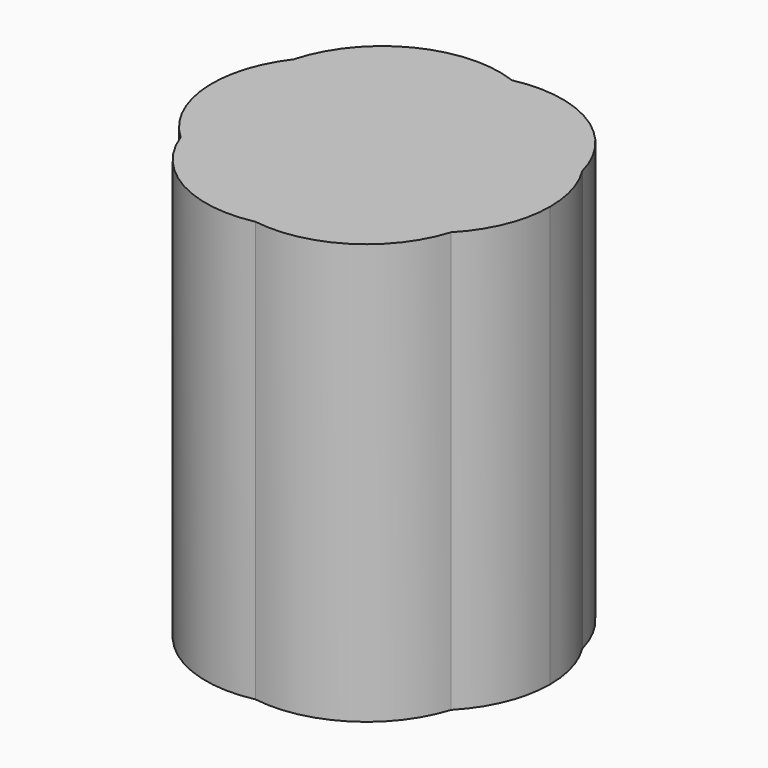
from build123d import *

# Parameters (mm, degrees)
F1_DEPTH = 5


with BuildPart() as f1:
    # F0 (on Top) → F1 (new body)
    with BuildSketch(Plane.XY):
        with BuildLine():
            ThreePointArc((-0.8988943353, -0.2747050753), (-0.8617178067, -0.0916116385), (-0.8492516278, 0.0948015993))
            ThreePointArc((-0.8492516278, 0.0948015993), (-0.8703764644, 0.3370892048), (-0.9331134618, 0.5720649731))
            ThreePointArc((-0.9331134618, 0.5720649731), (-1.2758447362, 0.8058613037), (-1.6720459361, 0.9289468827))
            ThreePointArc((-1.6720459361, 0.9289468827), (-2.0592079143, 0.785294631), (-2.3876180715, 0.5349406108))
            ThreePointArc((-2.3876180715, 0.5349406108), (-2.4494314254, 0.1540414271), (-2.4049112303, -0.2292639747))
            ThreePointArc((-2.4049112303, -0.2292639747), (-2.1066312225, -0.5672202335), (-1.7164187622, -0.7928740206))
            ThreePointArc((-1.7164187622, -0.7928740206), (-1.2614520098, -0.6066872767), (-0.8988943353, -0.2747050753))
        make_face()
        with BuildLine():
            ThreePointArc((-0.9331134618, 0.5720649731), (-0.8703764644, 0.3370892048), (-0.8492516278, 0.0948015993))
            ThreePointArc((-0.8492516278, 0.0948015993), (-0.8617178067, -0.0916116385), (-0.8988943353, -0.2747050753))
            ThreePointArc((-0.8988943353, -0.2747050753), (-0.7536616022, -0.0400351914), (-0.6572847743, 0.2185649019))
            ThreePointArc((-0.6572847743, 0.2185649019), (-0.7809552435, 0.4064291339), (-0.9331134618, 0.5720649731))
        make_face()
        with BuildLine():
            ThreePointArc((-1.6720459361, 0.9289468827), (-1.2758447362, 0.8058613037), (-0.9331134618, 0.5720649731))
            ThreePointArc((-0.9331134618, 0.5720649731), (-1.0180125198, 0.7611725612), (-1.1299043154, 0.9356711457))
            ThreePointArc((-1.1299043154, 0.9356711457), (-1.401303752, 0.9588044056), (-1.6720459361, 0.9289468827))
        make_face()
        with BuildLine():
            ThreePointArc((-1.1299043154, 0.9356711457), (-1.0180125198, 0.7611725612), (-0.9331134618, 0.5720649731))
            ThreePointArc((-0.9331134618, 0.5720649731), (-0.7809552435, 0.4064291339), (-0.6572847743, 0.2185649019))
            ThreePointArc((-0.6572847743, 0.2185649019), (-0.6225755838, 0.3956834749), (-0.6109413992, 0.5757955583))
            ThreePointArc((-0.6109413992, 0.5757955583), (-0.6131255758, 0.653967956), (-0.6196712903, 0.7318964362))
            ThreePointArc((-0.6196712903, 0.7318964362), (-0.8646934504, 0.8590591156), (-1.1299043154, 0.9356711457))
        make_face()
        with BuildLine():
            ThreePointArc((-0.6572847743, 0.2185649019), (-0.7536616022, -0.0400351914), (-0.8988943353, -0.2747050753))
            ThreePointArc((-0.8988943353, -0.2747050753), (-1.0346269029, -0.6013928976), (-1.2479146616, -0.8836278975))
            ThreePointArc((-1.2479146616, -0.8836278975), (-0.8622582937, -0.8374797639), (-0.5041231237, -0.6871478501))
            ThreePointArc((-0.5041231237, -0.6871478501), (-0.4895710534, -0.5713821921), (-0.4847091068, -0.4548068438))
            ThreePointArc((-0.4847091068, -0.4548068438), (-0.5285391201, -0.1072396313), (-0.6572847743, 0.2185649019))
        make_face()
        with BuildLine():
            ThreePointArc((-1.2479146616, -0.8836278975), (-1.0346269029, -0.6013928976), (-0.8988943353, -0.2747050753))
            ThreePointArc((-0.8988943353, -0.2747050753), (-1.2614520098, -0.6066872767), (-1.7164187622, -0.7928740206))
            ThreePointArc((-1.7164187622, -0.7928740206), (-1.4860620777, -0.858360236), (-1.2479146616, -0.8836278975))
        make_face()
        with BuildLine():
            ThreePointArc((-1.6720459361, 0.9289468827), (-1.401303752, 0.9588044056), (-1.1299043154, 0.9356711457))
            ThreePointArc((-1.1299043154, 0.9356711457), (-1.3763843902, 1.1893804158), (-1.678585825, 1.3732148899))
            ThreePointArc((-1.678585825, 1.3732148899), (-1.9737758003, 1.174153066), (-2.2092071036, 0.907067251))
            ThreePointArc((-2.2092071036, 0.907067251), (-1.9416866169, 0.944033234), (-1.6720459361, 0.9289468827))
        make_face()
        with BuildLine():
            ThreePointArc((-1.678585825, 1.3732148899), (-1.3763843902, 1.1893804158), (-1.1299043154, 0.9356711457))
            ThreePointArc((-1.1299043154, 0.9356711457), (-0.8646934504, 0.8590591156), (-0.6196712903, 0.7318964362))
            ThreePointArc((-0.6196712903, 0.7318964362), (-0.7361879783, 1.1545906135), (-0.9777387946, 1.5205137056))
            ThreePointArc((-0.9777387946, 1.5205137056), (-1.3377402962, 1.4924363094), (-1.678585825, 1.3732148899))
        make_face()
        with BuildLine():
            ThreePointArc((-0.6109413992, 0.5757955583), (-0.6225755838, 0.3956834749), (-0.6572847743, 0.2185649019))
            ThreePointArc((-0.6572847743, 0.2185649019), (-0.5285391201, -0.1072396313), (-0.4847091068, -0.4548068438))
            ThreePointArc((-0.4847091068, -0.4548068438), (-0.4895710534, -0.5713821921), (-0.5041231237, -0.6871478501))
            ThreePointArc((-0.5041231237, -0.6871478501), (-0.2236607638, -0.4676130058), (-0.0076714351, -0.1844111467))
            ThreePointArc((-0.0076714351, -0.1844111467), (-0.2197322329, 0.3364843866), (-0.6196712903, 0.7318964362))
            ThreePointArc((-0.6196712903, 0.7318964362), (-0.6131255758, 0.653967956), (-0.6109413992, 0.5757955583))
        make_face()
        with BuildLine():
            ThreePointArc((-2.3876180715, 0.5349406108), (-2.0592079143, 0.785294631), (-1.6720459361, 0.9289468827))
            ThreePointArc((-1.6720459361, 0.9289468827), (-1.9416866169, 0.944033234), (-2.2092071036, 0.907067251))
            ThreePointArc((-2.2092071036, 0.907067251), (-2.3121995682, 0.727613908), (-2.3876180715, 0.5349406108))
        make_face()
        with BuildLine():
            ThreePointArc((-0.5041231237, -0.6871478501), (-0.8622582937, -0.8374797639), (-1.2479146616, -0.8836278975))
            ThreePointArc((-1.2479146616, -0.8836278975), (-1.4228823891, -1.0352930345), (-1.6204555397, -1.1560443063))
            ThreePointArc((-1.6204555397, -1.1560443063), (-1.1797554002, -1.2715854362), (-0.7252917401, -1.2395051105))
            ThreePointArc((-0.7252917401, -1.2395051105), (-0.5850249567, -0.9752115997), (-0.5041231237, -0.6871478501))
        make_face()
        with BuildLine():
            ThreePointArc((-1.6204555397, -1.1560443063), (-1.4228823891, -1.0352930345), (-1.2479146616, -0.8836278975))
            ThreePointArc((-1.2479146616, -0.8836278975), (-1.4860620777, -0.858360236), (-1.7164187622, -0.7928740206))
            ThreePointArc((-1.7164187622, -0.7928740206), (-1.8987335129, -0.8197005507), (-2.0829923414, -0.822349163))
            ThreePointArc((-2.0829923414, -0.822349163), (-1.8688969211, -1.013000304), (-1.6204555397, -1.1560443063))
        make_face()
        with BuildLine():
            ThreePointArc((-2.0829923414, -0.822349163), (-1.8987335129, -0.8197005507), (-1.7164187622, -0.7928740206))
            ThreePointArc((-1.7164187622, -0.7928740206), (-2.1066312225, -0.5672202335), (-2.4049112303, -0.2292639747))
            ThreePointArc((-2.4049112303, -0.2292639747), (-2.2802207628, -0.5454928955), (-2.0829923414, -0.822349163))
        make_face()
        with BuildLine():
            ThreePointArc((-2.2092071036, 0.907067251), (-1.9737758003, 1.174153066), (-1.678585825, 1.3732148899))
            ThreePointArc((-1.678585825, 1.3732148899), (-1.9437880524, 1.461070974), (-2.2211544181, 1.4945196233))
            ThreePointArc((-2.2211544181, 1.4945196233), (-2.4678363793, 1.1504786171), (-2.600403435, 0.7484311329))
            ThreePointArc((-2.600403435, 0.7484311329), (-2.4108187653, 0.8425784603), (-2.2092071036, 0.907067251))
        make_face()
        with BuildLine():
            ThreePointArc((-2.2211544181, 1.4945196233), (-1.9437880524, 1.461070974), (-1.678585825, 1.3732148899))
            ThreePointArc((-1.678585825, 1.3732148899), (-1.3377402962, 1.4924363094), (-0.9777387946, 1.5205137056))
            ThreePointArc((-0.9777387946, 1.5205137056), (-1.2246565961, 1.7341375667), (-1.5143400889, 1.8847597055))
            ThreePointArc((-1.5143400889, 1.8847597055), (-1.8964893504, 1.7416981968), (-2.2211544181, 1.4945196233))
        make_face()
        with BuildLine():
            ThreePointArc((-0.9777387946, 1.5205137056), (-0.7361879783, 1.1545906135), (-0.6196712903, 0.7318964362))
            ThreePointArc((-0.6196712903, 0.7318964362), (-0.2197322329, 0.3364843866), (-0.0076714351, -0.1844111467))
            ThreePointArc((-0.0076714351, -0.1844111467), (0.1324037622, 0.153463889), (0.1801825481, 0.5160901266))
            ThreePointArc((0.1801825481, 0.5160901266), (0.1689176004, 0.6933327697), (0.1353040416, 0.8677230856))
            ThreePointArc((0.1353040416, 0.8677230856), (-0.3415262897, 1.3299959505), (-0.9777387946, 1.5205137056))
        make_face()
        with BuildLine():
            ThreePointArc((-2.3876180715, 0.5349406108), (-2.3121995682, 0.727613908), (-2.2092071036, 0.907067251))
            ThreePointArc((-2.2092071036, 0.907067251), (-2.4108187653, 0.8425784603), (-2.600403435, 0.7484311329))
            ThreePointArc((-2.600403435, 0.7484311329), (-2.6197629094, 0.5037322971), (-2.5960866966, 0.2594133531))
            ThreePointArc((-2.5960866966, 0.2594133531), (-2.5003846604, 0.4036326478), (-2.3876180715, 0.5349406108))
        make_face()
        with BuildLine():
            ThreePointArc((-2.4049112303, -0.2292639747), (-2.4494314254, 0.1540414271), (-2.3876180715, 0.5349406108))
            ThreePointArc((-2.3876180715, 0.5349406108), (-2.5003846604, 0.4036326478), (-2.5960866966, 0.2594133531))
            ThreePointArc((-2.5960866966, 0.2594133531), (-2.5235990735, 0.0060376947), (-2.4049112303, -0.2292639747))
        make_face()
        with BuildLine():
            ThreePointArc((-0.7252917401, -1.2395051105), (-1.1797554002, -1.2715854362), (-1.6204555397, -1.1560443063))
            ThreePointArc((-1.6204555397, -1.1560443063), (-2.0515783023, -1.2911728797), (-2.5032879922, -1.2819574666))
            ThreePointArc((-2.5032879922, -1.2819574666), (-2.103137308, -1.642235792), (-1.5966038505, -1.8248416468))
            ThreePointArc((-1.5966038505, -1.8248416468), (-1.1040138069, -1.6169233822), (-0.7252917401, -1.2395051105))
        make_face()
        with BuildLine():
            ThreePointArc((-2.5032879922, -1.2819574666), (-2.0515783023, -1.2911728797), (-1.6204555397, -1.1560443063))
            ThreePointArc((-1.6204555397, -1.1560443063), (-1.8688969211, -1.013000304), (-2.0829923414, -0.822349163))
            ThreePointArc((-2.0829923414, -0.822349163), (-2.443991306, -0.7555450361), (-2.7752107887, -0.5971887981))
            ThreePointArc((-2.7752107887, -0.5971887981), (-2.6851043864, -0.9577822288), (-2.5032879922, -1.2819574666))
        make_face()
        with BuildLine():
            ThreePointArc((-0.0076714351, -0.1844111467), (-0.2236607638, -0.4676130058), (-0.5041231237, -0.6871478501))
            ThreePointArc((-0.5041231237, -0.6871478501), (-0.5850249567, -0.9752115997), (-0.7252917401, -1.2395051105))
            ThreePointArc((-0.7252917401, -1.2395051105), (-0.3582467769, -1.0949100858), (-0.0461123451, -0.8536595467))
            ThreePointArc((-0.0461123451, -0.8536595467), (0.0004291531, -0.6497027944), (0.0160593202, -0.4410879202))
            ThreePointArc((0.0160593202, -0.4410879202), (0.0101140076, -0.3122022007), (-0.0076714351, -0.1844111467))
        make_face()
        with BuildLine():
            ThreePointArc((-2.0829923414, -0.822349163), (-2.2802207628, -0.5454928955), (-2.4049112303, -0.2292639747))
            ThreePointArc((-2.4049112303, -0.2292639747), (-2.5235990735, 0.0060376947), (-2.5960866966, 0.2594133531))
            ThreePointArc((-2.5960866966, 0.2594133531), (-2.7543003743, -0.1545319785), (-2.7752107887, -0.5971887981))
            ThreePointArc((-2.7752107887, -0.5971887981), (-2.443991306, -0.7555450361), (-2.0829923414, -0.822349163))
        make_face()
        with BuildLine():
            ThreePointArc((-2.600403435, 0.7484311329), (-2.4678363793, 1.1504786171), (-2.2211544181, 1.4945196233))
            ThreePointArc((-2.2211544181, 1.4945196233), (-2.8568261147, 1.3560919081), (-3.3612986917, 0.9453022329))
            ThreePointArc((-3.3612986917, 0.9453022329), (-3.4013148657, 0.4119003981), (-3.2383657317, -0.0975761874))
            ThreePointArc((-3.2383657317, -0.0975761874), (-3.0025129529, 0.3881134144), (-2.600403435, 0.7484311329))
        make_face()
        with BuildLine():
            ThreePointArc((-3.3612986917, 0.9453022329), (-2.8568261147, 1.3560919081), (-2.2211544181, 1.4945196233))
            ThreePointArc((-2.2211544181, 1.4945196233), (-1.8964893504, 1.7416981968), (-1.5143400889, 1.8847597055))
            ThreePointArc((-1.5143400889, 1.8847597055), (-2.6456617352, 1.8236457476), (-3.3612986917, 0.9453022329))
        make_face()
        with BuildLine():
            ThreePointArc((-1.5143400889, 1.8847597055), (-1.2246565961, 1.7341375667), (-0.9777387946, 1.5205137056))
            ThreePointArc((-0.9777387946, 1.5205137056), (-0.3415262897, 1.3299959505), (0.1353040416, 0.8677230856))
            ThreePointArc((0.1353040416, 0.8677230856), (-0.4851009384, 1.707808065), (-1.5143400889, 1.8847597055))
        make_face()
        with BuildLine():
            ThreePointArc((0.1801825481, 0.5160901266), (0.1324037622, 0.153463889), (-0.0076714351, -0.1844111467))
            ThreePointArc((-0.0076714351, -0.1844111467), (0.0101140076, -0.3122022007), (0.0160593202, -0.4410879202))
            ThreePointArc((0.0160593202, -0.4410879202), (0.0004291531, -0.6497027944), (-0.0461123451, -0.8536595467))
            ThreePointArc((-0.0461123451, -0.8536595467), (0.247351032, -0.4043432956), (0.3502102632, 0.1223689843))
            ThreePointArc((0.3502102632, 0.1223689843), (0.2954112314, 0.5102276636), (0.1353040416, 0.8677230856))
            ThreePointArc((0.1353040416, 0.8677230856), (0.1689176004, 0.6933327697), (0.1801825481, 0.5160901266))
        make_face()
        with BuildLine():
            ThreePointArc((-2.5960866966, 0.2594133531), (-2.6197629094, 0.5037322971), (-2.600403435, 0.7484311329))
            ThreePointArc((-2.600403435, 0.7484311329), (-3.0025129529, 0.3881134144), (-3.2383657317, -0.0975761874))
            ThreePointArc((-3.2383657317, -0.0975761874), (-3.037642018, -0.3759847941), (-2.7752107887, -0.5971887981))
            ThreePointArc((-2.7752107887, -0.5971887981), (-2.7543003743, -0.1545319785), (-2.5960866966, 0.2594133531))
        make_face()
        with BuildLine():
            ThreePointArc((-1.5966038505, -1.8248416468), (-2.103137308, -1.642235792), (-2.5032879922, -1.2819574666))
            ThreePointArc((-2.5032879922, -1.2819574666), (-2.8769397727, -1.1566006513), (-3.2008472728, -0.9320702176))
            ThreePointArc((-3.2008472728, -0.9320702176), (-2.5654977098, -1.6781329974), (-1.5966038505, -1.8248416468))
        make_face()
        with BuildLine():
            ThreePointArc((-3.2008472728, -0.9320702176), (-2.8769397727, -1.1566006513), (-2.5032879922, -1.2819574666))
            ThreePointArc((-2.5032879922, -1.2819574666), (-2.6851043864, -0.9577822288), (-2.7752107887, -0.5971887981))
            ThreePointArc((-2.7752107887, -0.5971887981), (-3.037642018, -0.3759847941), (-3.2383657317, -0.0975761874))
            ThreePointArc((-3.2383657317, -0.0975761874), (-3.2832962968, -0.5176866657), (-3.2008472728, -0.9320702176))
        make_face()
        with BuildLine():
            ThreePointArc((-0.0461123451, -0.8536595467), (-0.3582467769, -1.0949100858), (-0.7252917401, -1.2395051105))
            ThreePointArc((-0.7252917401, -1.2395051105), (-1.1040138069, -1.6169233822), (-1.5966038505, -1.8248416468))
            ThreePointArc((-1.5966038505, -1.8248416468), (-0.6407732495, -1.6275541737), (-0.0461123451, -0.8536595467))
        make_face()
        with BuildLine():
            ThreePointArc((-3.2383657317, -0.0975761874), (-3.4013148657, 0.4119003981), (-3.3612986917, 0.9453022329))
            ThreePointArc((-3.3612986917, 0.9453022329), (-3.6441663697, -0.0244161134), (-3.2008472728, -0.9320702176))
            ThreePointArc((-3.2008472728, -0.9320702176), (-3.2832962968, -0.5176866657), (-3.2383657317, -0.0975761874))
        make_face()
    extrude(amount=F1_DEPTH)


solid = f1.part
